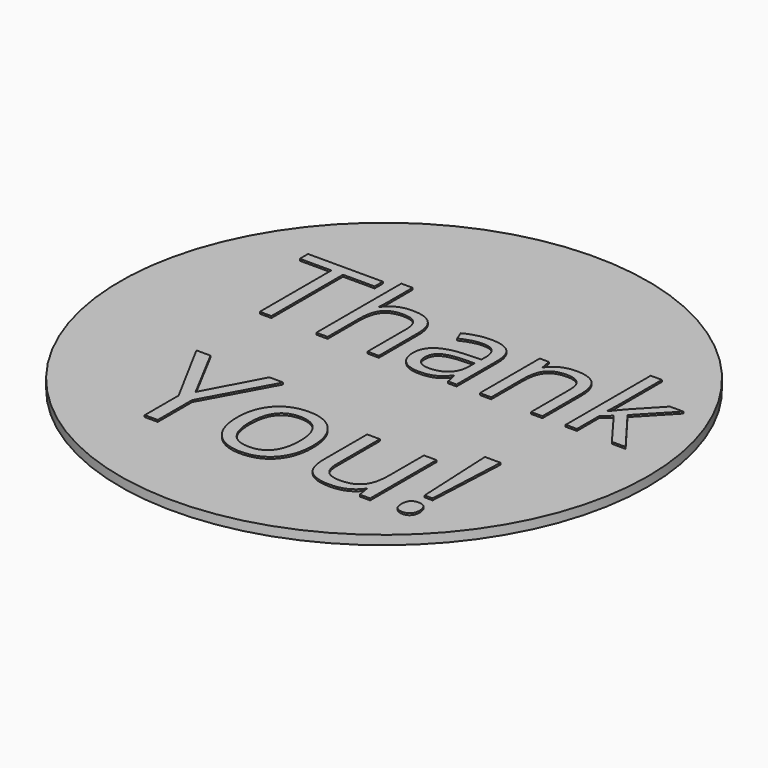
from build123d import *

# Parameters (mm, degrees)
F0_R         = 36.7600056066
F1_DEPTH     = 1.27
F2_TEXT_SIZE = 22.0133327982
F3_DEPTH     = 0.254
F4_TEXT_SIZE = 19.4733341535
F5_DEPTH     = 0.254
F6_TEXT_SIZE = 21.5899981817
F7_DEPTH     = 0.254


# Not quite as in the source:
# - Text() gives the source's letters only with a copy of the font that has no kerning and outlines rounded to 1/6400 em; it was checked with that copy


with BuildPart() as f1:
    # F0 (on Top) → F1 (new body)
    with BuildSketch(Plane.XY):
        Circle(F0_R)
    extrude(amount=F1_DEPTH)

    # F2 (on Top) → F3 (join)
    with BuildSketch(Plane.XY):
        with Locations((-31.9735735365, 0)):
            Text('Thank', F2_TEXT_SIZE, font='Open Sans', text_align=(TextAlign.LEFT, TextAlign.BOTTOM))
    extrude(amount=F3_DEPTH)

    # F4 (on face) → F5 (join)
    with BuildSketch(Plane.XY.offset(1.27)):
        with Locations((-24.6888007969, 3.5052001476)):
            Text('Thank', F4_TEXT_SIZE, font='Open Sans', text_align=(TextAlign.LEFT, TextAlign.BOTTOM))
    extrude(amount=F5_DEPTH)

    # F6 (on face) → F7 (join)
    with BuildSketch(Plane.XY.offset(1.27)):
        with Locations((-19.8120009154, -23.3171992004)):
            Text('You!', F6_TEXT_SIZE, font='Open Sans', text_align=(TextAlign.LEFT, TextAlign.BOTTOM))
    extrude(amount=F7_DEPTH)


solid = f1.part
